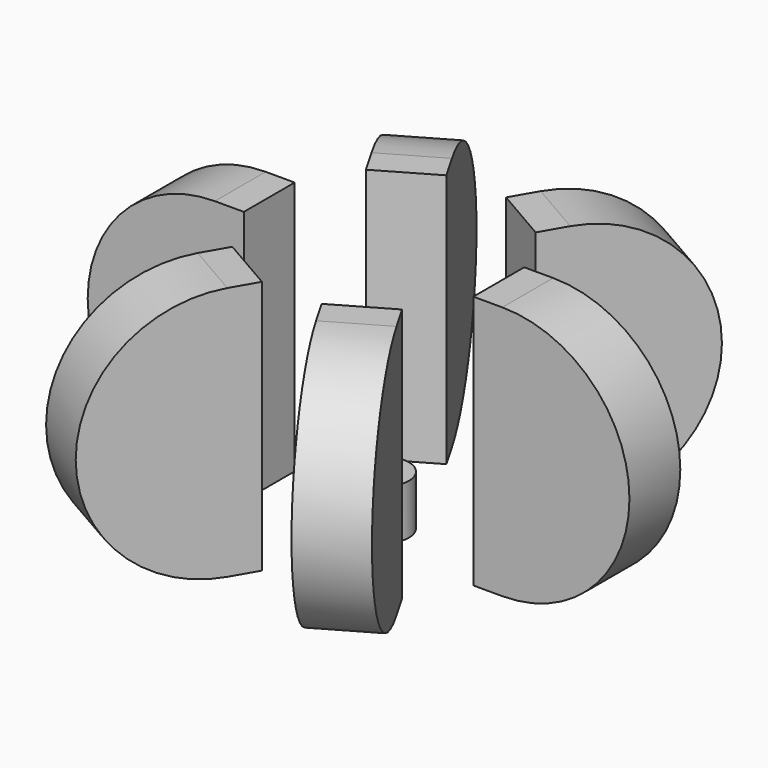
from build123d import *

# Parameters (mm, degrees)
F0_R            = 5
F1_DEPTH        = 10
F2_R            = 25.4
F2_R_2          = 5
F3_DEPTH        = 25.4
F5_DEPTH        = 6.35
F5_DEPTH_BACK   = 6.35
F5_COPIES_COUNT = 6


# Not quite as in the source:
# - a feature of the source that left no trace in its solid (it failed there, or was rolled back) is left out
# - a pattern or mirror of a feature is missing from the dataset's text; its kind, count and spacing are read off the source's solid


with BuildPart() as f1:
    # F0 (on Top) → F1 (new body)
    with BuildSketch(Plane.XY):
        Circle(F0_R)
    extrude(amount=F1_DEPTH)

    # F2 (on face) → F3 (cut)
    with BuildSketch(Plane(origin=(0, 0, 0), x_dir=(1, 0, 0), z_dir=(0, 0, -1))):
        Circle(F2_R)
        Circle(F2_R_2, mode=Mode.SUBTRACT)
    extrude(amount=-F3_DEPTH, mode=Mode.SUBTRACT)


with BuildPart() as f5:
    # F4 (on Front) → F5 (new body, two sides)
    with BuildSketch(Plane.XZ) as f5_sk:
        with BuildLine():
            ThreePointArc((-28.718591857, 50.8), (-54.118591857, 25.4), (-28.718591857, 0))
            Line((-28.718591857, 0), (-22.9244896994, 0))
            Line((-22.9244896994, 0), (-22.9244896994, 50.8))
            Line((-22.9244896994, 50.8), (-28.718591857, 50.8))
        make_face()
    extrude(amount=F5_DEPTH)
    extrude(f5_sk.sketch, amount=-F5_DEPTH_BACK)


with BuildPart() as f5_copies_1:
    # F5_copies: instance of F5
    add(f5.part.rotate(Axis((0, 0, 0), (0, 0, 1)), 1 * 360 / F5_COPIES_COUNT))


with BuildPart() as f5_copies_2:
    # F5_copies: instance of F5
    add(f5.part.rotate(Axis((0, 0, 0), (0, 0, 1)), 2 * 360 / F5_COPIES_COUNT))


with BuildPart() as f5_copies_3:
    # F5_copies: instance of F5
    add(f5.part.rotate(Axis((0, 0, 0), (0, 0, 1)), 3 * 360 / F5_COPIES_COUNT))


with BuildPart() as f5_copies_4:
    # F5_copies: instance of F5
    add(f5.part.rotate(Axis((0, 0, 0), (0, 0, 1)), 4 * 360 / F5_COPIES_COUNT))


with BuildPart() as f5_copies_5:
    # F5_copies: instance of F5
    add(f5.part.rotate(Axis((0, 0, 0), (0, 0, 1)), 5 * 360 / F5_COPIES_COUNT))


solid = Compound([f1.part, f5.part, f5_copies_1.part, f5_copies_2.part, f5_copies_3.part, f5_copies_4.part, f5_copies_5.part])
